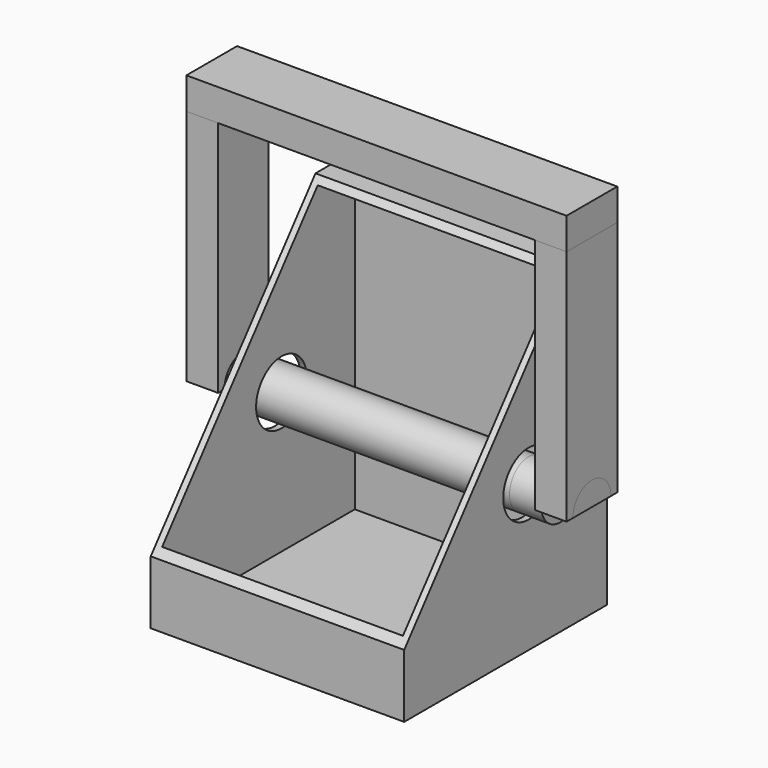
from build123d import *

# Parameters (mm, degrees)
F1_DEPTH  = 101.6
F2_T      = -2.54
F3_R      = 12.7
F4_DEPTH  = 101.6
F5_R      = 9.525
F6_DEPTH  = 114.3
F7_DEPTH  = 12.7
F9_DEPTH  = 12.7
F11_DEPTH = 12.7
F13_DEPTH = 12.7
F15_DEPTH = 12.7
F17_DEPTH = 25.4


with BuildPart() as f1:
    # F0 (on Right) → F1 (new body)
    with BuildSketch(Plane.YZ):
        Polygon((0, 25.4), (0, 0), (101.6, 0), (101.6, 127), (82.55, 127), align=None)
    extrude(amount=-F1_DEPTH)

    # F2
    f2_openings = [f1.faces().sort_by_distance(p)[0] for p in [
        (-50.8, 41.275, 76.2),
    ]]
    offset(amount=F2_T, openings=f2_openings)

    # F3 (on face) → F4 (cut)
    with BuildSketch(Plane.YZ):
        with Locations((62.3146630824, 58.7586686015)):
            Circle(F3_R)
    extrude(amount=-F4_DEPTH, mode=Mode.SUBTRACT)


with BuildPart() as f6:
    # F5 (on face) → F6 (new body)
    with BuildSketch(Plane.YZ):
        with Locations((62.3146630824, 58.7586686015)):
            Circle(F5_R)
    extrude(amount=-F6_DEPTH)

    # F7 (add): a face of the model
    f7_faces = [f6.faces().sort_by_distance(p)[0] for p in [
        (0, 62.3146630824, 58.7586686015),
    ]]
    extrude(f7_faces, amount=F7_DEPTH)


with BuildPart() as f9:
    # F8 (on face) → F9 (new body)
    with BuildSketch(Plane.YZ.offset(12.7)):
        with BuildLine():
            ThreePointArc((52.7896630824, 58.7586686015), (62.3146630824, 68.2836686015), (71.8396630824, 58.7586686015))
            Line((71.8396630824, 58.7586686015), (75.0146630824, 58.7586686015))
            Line((75.0146630824, 58.7586686015), (75.0146630824, 154.0086686015))
            Line((75.0146630824, 154.0086686015), (49.6146630824, 154.0086686015))
            Line((49.6146630824, 154.0086686015), (49.6146630824, 58.7586686015))
            Line((49.6146630824, 58.7586686015), (52.7896630824, 58.7586686015))
        make_face()
    extrude(amount=F9_DEPTH)


with BuildPart() as f11:
    # F10 (on face) → F11 (new body)
    with BuildSketch(Plane.YZ.offset(12.7)):
        with BuildLine():
            ThreePointArc((71.8396630824, 58.7586686015), (62.3096746028, 68.2836672952), (52.7896683075, 58.7486916438))
            Line((52.7896683075, 58.7486916438), (71.8396578572, 58.7486916438))
            ThreePointArc((71.8396578572, 58.7486916438), (71.8396617761, 58.7536801219), (71.8396630824, 58.7586686015))
        make_face()
    extrude(amount=F11_DEPTH)


with BuildPart() as f13:
    # F12 (on face) → F13 (new body)
    with BuildSketch(Plane(origin=(-114.3, 0, 0), x_dir=(0, -1, 0), z_dir=(-1, 0, 0))):
        with BuildLine():
            ThreePointArc((-71.8396630824, 58.7586686015), (-62.3146630824, 68.2836686015), (-52.7896630824, 58.7586686015))
            Line((-52.7896630824, 58.7586686015), (-49.6146630824, 58.7586686015))
            Line((-49.6146630824, 58.7586686015), (-49.6146630824, 154.0086686015))
            Line((-49.6146630824, 154.0086686015), (-75.003027916, 154.0086686015))
            Line((-75.003027916, 154.0086686015), (-75.003027916, 58.7586686015))
            Line((-75.003027916, 58.7586686015), (-71.8396630824, 58.7586686015))
        make_face()
    extrude(amount=F13_DEPTH)


with BuildPart() as f15:
    # F14 (on face) → F15 (new body)
    with BuildSketch(Plane(origin=(-114.3, 0, 0), x_dir=(0, -1, 0), z_dir=(-1, 0, 0))):
        with BuildLine():
            Line((-71.8396630824, 58.7586686015), (-62.3146630824, 58.7586686015))
            Line((-62.3146630824, 58.7586686015), (-52.7896630824, 58.7586686015))
            ThreePointArc((-52.7896630824, 58.7586686015), (-62.3146630824, 68.2836686015), (-71.8396630824, 58.7586686015))
        make_face()
    extrude(amount=F15_DEPTH)


with BuildPart() as f17:
    # F16 (on face) → F17 (new body)
    with BuildSketch(Plane.XZ.offset(-49.6146630824)):
        Polygon((-127, 166.7086686015), (-127, 154.0086686015), (-114.3, 154.0086686015), (25.4, 154.0086686015), (25.4, 166.7086686015), align=None)
    extrude(amount=-F17_DEPTH)


solid = Compound([f1.part, f6.part, f9.part, f11.part, f13.part, f15.part, f17.part])
